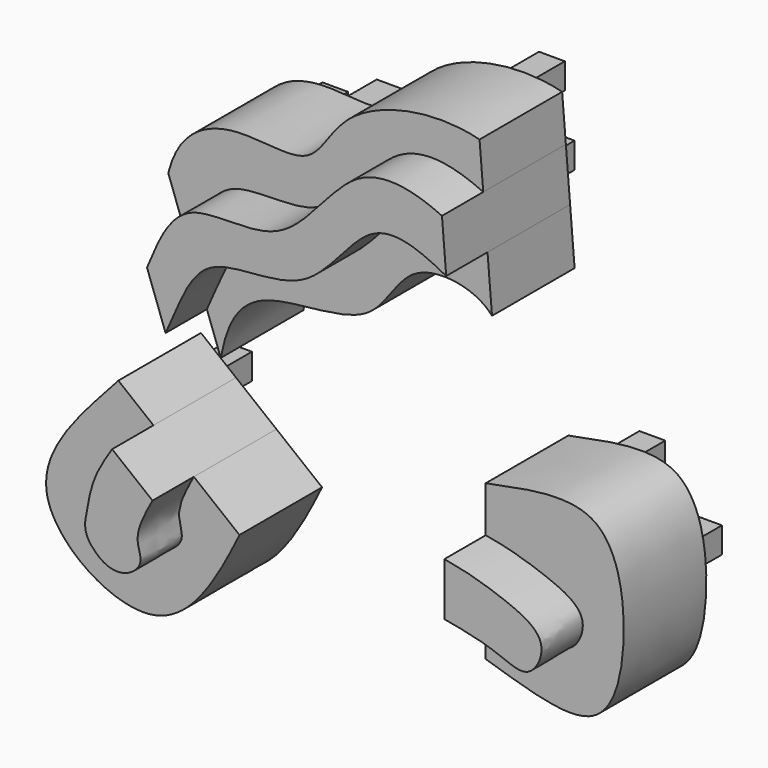
from build123d import *

# Parameters (mm, degrees)
F1_W     = 6.35
F1_H     = 6.35
F2_DEPTH = 38.1
F1_H_2   = 6.3500067535
F1_W_2   = 6.3500067535
F3_DEPTH = 25.4
F5_DEPTH = 12.7


with BuildPart() as f2:
    # F1 (on Front) → F2 (new body)
    with BuildSketch(Plane.XZ):
        with Locations((-40.2297045912, -38.3458063006)):
            Rectangle(F1_W, F1_H)
    extrude(amount=F2_DEPTH)


with BuildPart() as f2b:
    # F1 (on Front) → F2, piece 2 (new body)
    with BuildSketch(Plane.XZ):
        with Locations((-37.0547045912, -18.8041891663)):
            Rectangle(F1_W, F1_H_2)
    extrude(amount=F2_DEPTH)


with BuildPart() as f2c:
    # F1 (on Front) → F2, piece 3 (new body)
    with BuildSketch(Plane.XZ):
        with Locations((-23.0328589304, -41.5208063006)):
            Rectangle(F1_W, F1_H)
    extrude(amount=F2_DEPTH)


with BuildPart() as f2d:
    # F1 (on Front) → F2, piece 4 (new body)
    with BuildSketch(Plane.XZ):
        with Locations((-10.0376270711, 25.8038714528)):
            Rectangle(F1_W, F1_H)
    extrude(amount=F2_DEPTH)


with BuildPart() as f2e:
    # F1 (on Front) → F2, piece 5 (new body)
    with BuildSketch(Plane.XZ):
        with Locations((-13.3560132235, 45.1611280441)):
            Rectangle(F1_W, F1_H)
    extrude(amount=F2_DEPTH)


with BuildPart() as f2f:
    # F1 (on Front) → F2, piece 6 (new body)
    with BuildSketch(Plane.XZ):
        with Locations((0, 33.6901598692)):
            Rectangle(F1_W, F1_H)
    extrude(amount=F2_DEPTH)


with BuildPart() as f2g:
    # F1 (on Front) → F2, piece 7 (new body)
    with BuildSketch(Plane.XZ):
        with Locations((0, 50.138708204)):
            Rectangle(F1_W, F1_H)
    extrude(amount=F2_DEPTH)


with BuildPart() as f2h:
    # F1 (on Front) → F2, piece 8 (new body)
    with BuildSketch(Plane.XZ):
        with Locations((14.2972143367, 36.8651598692)):
            Rectangle(F1_W_2, F1_H)
    extrude(amount=F2_DEPTH)


with BuildPart() as f2i:
    # F1 (on Front) → F2, piece 9 (new body)
    with BuildSketch(Plane.XZ):
        with Locations((15.0551136671, 51.7979040742)):
            Rectangle(F1_W_2, F1_H)
    extrude(amount=F2_DEPTH)


with BuildPart() as f2j:
    # F1 (on Front) → F2, piece 10 (new body)
    with BuildSketch(Plane.XZ):
        with Locations((25.91156587, 62.1217750013)):
            Rectangle(F1_W, F1_H)
    extrude(amount=F2_DEPTH)


with BuildPart() as f2k:
    # F1 (on Front) → F2, piece 11 (new body)
    with BuildSketch(Plane.XZ):
        with Locations((27.7551170439, 43.5019358993)):
            Rectangle(F1_W, F1_H)
    extrude(amount=F2_DEPTH)


with BuildPart() as f2l:
    # F1 (on Front) → F2, piece 12 (new body)
    with BuildSketch(Plane.XZ):
        with Locations((42.3191487789, 52.7196787298)):
            Rectangle(F1_W, F1_H)
    extrude(amount=F2_DEPTH)


with BuildPart() as f2m:
    # F1 (on Front) → F2, piece 13 (new body)
    with BuildSketch(Plane.XZ):
        with Locations((39.9225354195, 69.1272616386)):
            Rectangle(F1_W, F1_H)
    extrude(amount=F2_DEPTH)


with BuildPart() as f2n:
    # F1 (on Front) → F2, piece 14 (new body)
    with BuildSketch(Plane.XZ):
        with Locations((64.626082778, -4.9833874218)):
            Rectangle(F1_W, F1_H)
    extrude(amount=F2_DEPTH)


with BuildPart() as f2o:
    # F1 (on Front) → F2, piece 15 (new body)
    with BuildSketch(Plane.XZ):
        with Locations((78.5702839494, -18.804192543)):
            Rectangle(F1_W, F1_H)
    extrude(amount=F2_DEPTH)


with BuildPart() as f2p:
    # F1 (on Front) → F2, piece 16 (new body)
    with BuildSketch(Plane.XZ):
        with Locations((62.9001185298, -27.6532266289)):
            Rectangle(F1_W, F1_H)
    extrude(amount=F2_DEPTH)


with BuildPart() as f2q:
    # F0 (on Front) → F2, piece 17 (new body)
    with BuildSketch(Plane.XZ):
        with BuildLine():
            Line((-17.6866312354, -21.9644817992), (-27.6188283527, -14.0498459629))
            add(Edge.make_bspline(
                [(-34.2003328863, -31.4649609791), (-33.7270573, -28.4063929308), (-32.4419022716, -21.233363344), (-29.2826732849, -16.6660639516), (-27.6188283527, -14.0498459629)],
                knots=[0.193358709, 0.193358709, 0.193358709, 0.193358709, 0.5445747797, 1, 1, 1, 1], degree=3))
            ThreePointArc((-34.2003328863, -31.4649609791), (-33.9356816121, -34.4840111506), (-32.3019141327, -37.0365604758))
            add(Edge.make_bspline(
                [(-32.3019141327, -37.0365604758), (-27.5338690011, -42.4975869781), (-18.3358657112, -37.5704930349), (-22.9948761498, -31.3972228752), (-19.2179106721, -24.7697868671), (-17.6866312354, -21.9644817992)],
                knots=[0, 0, 0, 0, 0.3777187462, 0.6425151646, 1, 1, 1, 1], degree=3))
        make_face()
    extrude(amount=F2_DEPTH)


with BuildPart() as f2r:
    # F0 (on Front) → F2, piece 18 (new body)
    with BuildSketch(Plane.XZ):
        with BuildLine():
            add(Edge.make_bspline(
                [(-19.0486874526, 28.069653114), (-16.1297544348, 35.2400638352), (-10.5658538677, 47.9792316154), (15.9764685433, 40.6875166992), (30.6201312255, 69.2760269626), (46.2685888311, 66.224880626), (53.512246195, 62.8631052811)],
                knots=[0, 0, 0, 0, 0.2330057974, 0.4807241751, 0.7563605987, 1, 1, 1, 1], degree=3))
            Line((-19.0486874526, 28.069653114), (-14.4754832667, 15.369653114))
            add(Edge.make_bspline(
                [(-14.4754832667, 15.369653114), (-11.0304212691, 22.7301711692), (-6.5915277564, 38.1114839776), (21.6735434079, 32.2299303201), (34.9649145222, 59.0130925658), (48.2982864129, 53.5396952684), (54.5598767881, 50.1631052811)],
                knots=[0, 0, 0, 0, 0.2480530731, 0.5061702778, 0.770560426, 1, 1, 1, 1], degree=3))
            Line((54.5598767881, 50.1631052811), (53.512246195, 62.8631052811))
        make_face()
    extrude(amount=F2_DEPTH)


with BuildPart() as f2s:
    # F0 (on Front) → F2, piece 19 (new body)
    with BuildSketch(Plane.XZ):
        with BuildLine():
            add(Edge.make_bspline(
                [(54.1254356503, -11.2661298692), (59.7488794797, -12.2260240818), (67.5823607362, -14.5945214976), (80.585444218, -20.1439584301), (74.8881350786, -32.0013198048), (67.0493091554, -26.4798312578), (56.1887574918, -24.6968010149), (54.1254356503, -24.2915211687)],
                knots=[0, 0, 0, 0, 0.2187280918, 0.4089489976, 0.5670249139, 0.7515180354, 0.8867481159, 0.8867481159, 0.8867481159, 0.8867481159], degree=3))
            Line((54.1254356503, -11.2661298692), (54.1254356503, -23.9464010264))
            add(Edge.make_bspline(
                [(54.1254356503, -23.9464010264), (54.1827755841, -23.9515000065), (54.1927046668, -23.9583031719), (54.1254356503, -23.9661298692)],
                knots=[0.9859989499, 0.9859989499, 0.9859989499, 0.9859989499, 1, 1, 1, 1], degree=3))
            Line((54.1254356503, -23.9661298692), (54.1254356503, -24.2915211687))
        make_face()
    extrude(amount=F2_DEPTH)


with BuildPart() as f3:
    # F0 (on Front) → F3 (new body)
    with BuildSketch(Plane.XZ):
        with BuildLine():
            Line((-27.6188283527, -14.0498459629), (-36.2524676494, -7.1699874413))
            add(Edge.make_bspline(
                [(-36.2524676494, -7.1699874413), (-44.3601298649, -16.3127867262), (-66.2621910158, -37.3400432047), (-25.0597181498, -65.3858457354), (-12.5465969567, -43.3326320743), (-6.4558762973, -30.9138949504)],
                knots=[0, 0, 0, 0, 0.3437425818, 0.6646535352, 1, 1, 1, 1], degree=3))
            Line((-6.4558762973, -30.9138949504), (-17.6866312354, -21.9644817992))
            add(Edge.make_bspline(
                [(-32.3019141327, -37.0365604758), (-27.5338690011, -42.4975869781), (-18.3358657112, -37.5704930349), (-22.9948761498, -31.3972228752), (-19.2179106721, -24.7697868671), (-17.6866312354, -21.9644817992)],
                knots=[0, 0, 0, 0, 0.3777187462, 0.6425151646, 1, 1, 1, 1], degree=3))
            ThreePointArc((-32.3019141327, -37.0365604758), (-33.9356816121, -34.4840111506), (-34.2003328863, -31.4649609791))
            add(Edge.make_bspline(
                [(-34.2003328863, -31.4649609791), (-33.7270573, -28.4063929308), (-32.4419022716, -21.233363344), (-29.2826732849, -16.6660639516), (-27.6188283527, -14.0498459629)],
                knots=[0.193358709, 0.193358709, 0.193358709, 0.193358709, 0.5445747797, 1, 1, 1, 1], degree=3))
        make_face()
    extrude(amount=F3_DEPTH)


with BuildPart() as f3b:
    # F0 (on Front) → F3, piece 2 (new body)
    with BuildSketch(Plane.XZ):
        with BuildLine():
            add(Edge.make_bspline(
                [(-23.9825686231, 41.7712698178), (-21.4420531824, 52.006544319), (-8.4671105715, 58.7834854613), (12.1191314916, 52.7538064445), (18.2112189001, 71.7317265194), (40.9638800917, 76.9343210212), (52.5984480654, 73.9407087061)],
                knots=[0, 0, 0, 0, 0.2533810693, 0.478458636, 0.6910852846, 1, 1, 1, 1], degree=3))
            Line((-23.9825686231, 41.7712698178), (-19.0486874526, 28.069653114))
            add(Edge.make_bspline(
                [(-19.0486874526, 28.069653114), (-16.1297544348, 35.2400638352), (-10.5658538677, 47.9792316154), (15.9764685433, 40.6875166992), (30.6201312255, 69.2760269626), (46.2685888311, 66.224880626), (53.512246195, 62.8631052811)],
                knots=[0, 0, 0, 0, 0.2330057974, 0.4807241751, 0.7563605987, 1, 1, 1, 1], degree=3))
            Line((53.512246195, 62.8631052811), (52.5984480654, 73.9407087061))
        make_face()
    extrude(amount=F3_DEPTH)


with BuildPart() as f3c:
    # F0 (on Front) → F3, piece 3 (new body)
    with BuildSketch(Plane.XZ):
        with BuildLine():
            add(Edge.make_bspline(
                [(-14.4754832667, 15.369653114), (-11.0304212691, 22.7301711692), (-6.5915277564, 38.1114839776), (21.6735434079, 32.2299303201), (34.9649145222, 59.0130925658), (48.2982864129, 53.5396952684), (54.5598767881, 50.1631052811)],
                knots=[0, 0, 0, 0, 0.2480530731, 0.5061702778, 0.770560426, 1, 1, 1, 1], degree=3))
            Line((-14.4754832667, 15.369653114), (-11.0743479794, 5.9245427732))
            add(Edge.make_bspline(
                [(-11.0743479794, 5.9245427732), (-9.4445674212, 14.7705738075), (-2.7073950203, 25.5037827375), (27.8344009391, 22.4919113192), (33.8434578857, 44.1681388725), (51.7471545308, 41.3619016171), (55.6664453235, 36.7486245534)],
                knots=[0, 0, 0, 0, 0.2454263123, 0.5247406445, 0.7594550303, 0.9986831478, 0.9986831478, 0.9986831478, 0.9986831478], degree=3))
            Line((55.6664453235, 36.7486245534), (54.5598767881, 50.1631052811))
        make_face()
    extrude(amount=F3_DEPTH)


with BuildPart() as f3d:
    # F0 (on Front) → F3, piece 4 (new body)
    with BuildSketch(Plane.XZ):
        with BuildLine():
            add(Edge.make_bspline(
                [(54.1254356503, 0), (65.550894041, 2.2950380582), (85.1356443712, 6.4373789311), (89.8562946989, -23.1933867721), (83.3322430853, -47.6878586823), (65.211646282, -41.5107788404), (54.1254356503, -38.1)],
                knots=[0, 0, 0, 0, 0.2641645516, 0.5127620774, 0.7380533567, 1, 1, 1, 1], degree=3))
            Line((54.1254356503, 0), (54.1254356503, -11.2661298692))
            add(Edge.make_bspline(
                [(54.1254356503, -11.2661298692), (59.7488794797, -12.2260240818), (67.5823607362, -14.5945214976), (80.585444218, -20.1439584301), (74.8881350786, -32.0013198048), (67.0493091554, -26.4798312578), (56.1887574918, -24.6968010149), (54.1254356503, -24.2915211687)],
                knots=[0, 0, 0, 0, 0.2187280918, 0.4089489976, 0.5670249139, 0.7515180354, 0.8867481159, 0.8867481159, 0.8867481159, 0.8867481159], degree=3))
            Line((54.1254356503, -24.2915211687), (54.1254356503, -38.1))
        make_face()
    extrude(amount=F3_DEPTH)


with BuildPart() as f3e:
    # F0 (on Front) → F3, piece 5 (new body)
    with BuildSketch(Plane.XZ):
        with BuildLine():
            Line((54.1254356503, -23.9661298692), (54.1254356503, -23.9464010264))
            add(Edge.make_bspline(
                [(54.1254356503, -24.2915211687), (53.2596440999, -24.1214614817), (52.5245292939, -23.9314515009), (53.9513529163, -23.9309206387), (54.1254356503, -23.9464010264)],
                knots=[0.8867481159, 0.8867481159, 0.8867481159, 0.8867481159, 0.9434920803, 0.9859989499, 0.9859989499, 0.9859989499, 0.9859989499], degree=3))
            Line((54.1254356503, -24.2915211687), (54.1254356503, -23.9661298692))
        make_face()
    extrude(amount=F3_DEPTH)


with BuildPart() as f5:
    # F1 (on Front) → F5 (new body)
    with BuildSketch(Plane.XZ):
        with Locations((-40.2297045912, -38.3458063006)):
            Rectangle(F1_W, F1_H)
    extrude(amount=-F5_DEPTH)


with BuildPart() as f5b:
    # F1 (on Front) → F5, piece 2 (new body)
    with BuildSketch(Plane.XZ):
        with Locations((-37.0547045912, -18.8041891663)):
            Rectangle(F1_W, F1_H_2)
    extrude(amount=-F5_DEPTH)


with BuildPart() as f5c:
    # F1 (on Front) → F5, piece 3 (new body)
    with BuildSketch(Plane.XZ):
        with Locations((-23.0328589304, -41.5208063006)):
            Rectangle(F1_W, F1_H)
    extrude(amount=-F5_DEPTH)


with BuildPart() as f5d:
    # F1 (on Front) → F5, piece 4 (new body)
    with BuildSketch(Plane.XZ):
        with Locations((-10.0376270711, 25.8038714528)):
            Rectangle(F1_W, F1_H)
    extrude(amount=-F5_DEPTH)


with BuildPart() as f5e:
    # F1 (on Front) → F5, piece 5 (new body)
    with BuildSketch(Plane.XZ):
        with Locations((-13.3560132235, 45.1611280441)):
            Rectangle(F1_W, F1_H)
    extrude(amount=-F5_DEPTH)


with BuildPart() as f5f:
    # F1 (on Front) → F5, piece 6 (new body)
    with BuildSketch(Plane.XZ):
        with Locations((0, 33.6901598692)):
            Rectangle(F1_W, F1_H)
    extrude(amount=-F5_DEPTH)


with BuildPart() as f5g:
    # F1 (on Front) → F5, piece 7 (new body)
    with BuildSketch(Plane.XZ):
        with Locations((0, 50.138708204)):
            Rectangle(F1_W, F1_H)
    extrude(amount=-F5_DEPTH)


with BuildPart() as f5h:
    # F1 (on Front) → F5, piece 8 (new body)
    with BuildSketch(Plane.XZ):
        with Locations((14.2972143367, 36.8651598692)):
            Rectangle(F1_W_2, F1_H)
    extrude(amount=-F5_DEPTH)


with BuildPart() as f5i:
    # F1 (on Front) → F5, piece 9 (new body)
    with BuildSketch(Plane.XZ):
        with Locations((15.0551136671, 51.7979040742)):
            Rectangle(F1_W_2, F1_H)
    extrude(amount=-F5_DEPTH)


with BuildPart() as f5j:
    # F1 (on Front) → F5, piece 10 (new body)
    with BuildSketch(Plane.XZ):
        with Locations((25.91156587, 62.1217750013)):
            Rectangle(F1_W, F1_H)
    extrude(amount=-F5_DEPTH)


with BuildPart() as f5k:
    # F1 (on Front) → F5, piece 11 (new body)
    with BuildSketch(Plane.XZ):
        with Locations((27.7551170439, 43.5019358993)):
            Rectangle(F1_W, F1_H)
    extrude(amount=-F5_DEPTH)


with BuildPart() as f5l:
    # F1 (on Front) → F5, piece 12 (new body)
    with BuildSketch(Plane.XZ):
        with Locations((42.3191487789, 52.7196787298)):
            Rectangle(F1_W, F1_H)
    extrude(amount=-F5_DEPTH)


with BuildPart() as f5m:
    # F1 (on Front) → F5, piece 13 (new body)
    with BuildSketch(Plane.XZ):
        with Locations((39.9225354195, 69.1272616386)):
            Rectangle(F1_W, F1_H)
    extrude(amount=-F5_DEPTH)


with BuildPart() as f5n:
    # F1 (on Front) → F5, piece 14 (new body)
    with BuildSketch(Plane.XZ):
        with Locations((64.626082778, -4.9833874218)):
            Rectangle(F1_W, F1_H)
    extrude(amount=-F5_DEPTH)


with BuildPart() as f5o:
    # F1 (on Front) → F5, piece 15 (new body)
    with BuildSketch(Plane.XZ):
        with Locations((78.5702839494, -18.804192543)):
            Rectangle(F1_W, F1_H)
    extrude(amount=-F5_DEPTH)


with BuildPart() as f5p:
    # F1 (on Front) → F5, piece 16 (new body)
    with BuildSketch(Plane.XZ):
        with Locations((62.9001185298, -27.6532266289)):
            Rectangle(F1_W, F1_H)
    extrude(amount=-F5_DEPTH)


solid = Compound([f2q.part, f2r.part, f2s.part, f3.part, f3b.part, f3c.part, f3d.part, f3e.part, f5.part, f5b.part, f5c.part, f5d.part, f5e.part, f5f.part, f5g.part, f5h.part, f5i.part, f5j.part, f5k.part, f5l.part, f5m.part, f5n.part, f5o.part, f5p.part])
